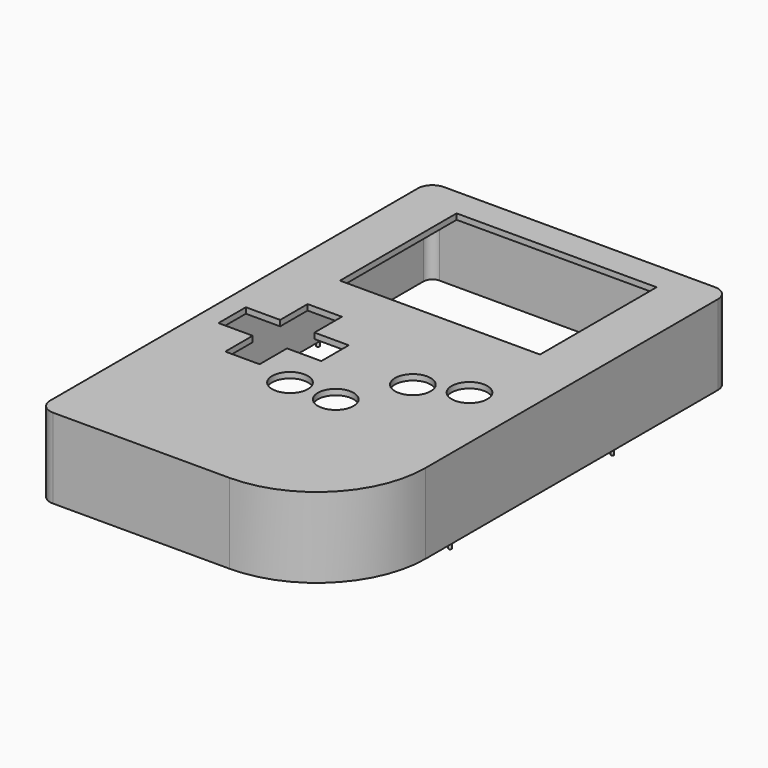
from build123d import *

# Parameters (mm, degrees)
F0_W         = 105
F0_H         = 171
F1_DEPTH     = 28
F3_R         = 38.1
F4_R         = 5.08
F5_T         = -2
F2_W         = 70
F2_H         = 51
F2_R         = 6.25
F6_DEPTH     = 2
F7_TEXT_SIZE = 7.9061016953
F8_DEPTH     = 1
F9_R         = 0.5
F10_DEPTH    = 2


# Not quite as in the source:
# - Text() gives the source's letters only with a copy of the font that has no kerning and outlines rounded to 1/6400 em; it was checked with that copy


with BuildPart() as f1:
    # F0 (on Top) → F1 (new body)
    with BuildSketch(Plane.XY):
        with Locations((52.5, 85.5)):
            Rectangle(F0_W, F0_H)
    extrude(amount=F1_DEPTH)

    # F3
    f3_edges = [f1.edges().sort_by_distance(p)[0] for p in [
        (105, 0, 14),
    ]]
    fillet(f3_edges, radius=F3_R)

    # F4
    f4_edges = [f1.edges().sort_by_distance(p)[0] for p in [
        (0, 0, 14),
        (0, 171, 14),
        (105, 171, 14),
    ]]
    fillet(f4_edges, radius=F4_R)

    # F5
    f5_openings = [f1.faces().sort_by_distance(p)[0] for p in [
        (51.738712, 86.834126, 0),
    ]]
    offset(amount=F5_T, openings=f5_openings)

    # F2 (on face) → F6 (cut, through all)
    with BuildSketch(Plane.XY.offset(28)):
        with Locations((52.5, 135.5)):
            Rectangle(F2_W, F2_H)
        Polygon((19.25, 81.6398638973), (7.25, 81.6398638973), (7.25, 69.6398638973), (19.25, 69.6398638973), (19.25, 57.6398638973), (31.25, 57.6398638973), (31.25, 69.6398638973), (43.25, 69.6398638973), (43.25, 81.6398638973), (31.25, 81.6398638973), (31.25, 93.6398638973), (19.25, 93.6398638973), align=None)
        with Locations((86.5, 80.3898638973)):
            Circle(F2_R)
        with Locations((71.5, 74.3898638973)):
            Circle(F2_R)
        with Locations((44.5, 54.3898638973)):
            Circle(F2_R)
        with Locations((60.5, 54.3898638973)):
            Circle(F2_R)
    extrude(amount=-F6_DEPTH, mode=Mode.SUBTRACT)

    # F7 (on face) → F8 (cut)
    with BuildSketch(Plane(origin=(0, 0, 26), x_dir=(1, 0, 0), z_dir=(0, 0, -1))):
        with Locations((2, -18.2658384198)):
            Text('Jane is rad', F7_TEXT_SIZE, font='Arimo', text_align=(TextAlign.LEFT, TextAlign.BOTTOM))
    extrude(amount=-F8_DEPTH, mode=Mode.SUBTRACT)

    # F9 (on face) → F10 (join)
    with BuildSketch(Plane.XY):
        with Locations((104, 50)):
            Circle(F9_R)
        with Locations((1, 50)):
            Circle(F9_R)
        with Locations((1, 121)):
            Circle(F9_R)
        with Locations((104, 121)):
            Circle(F9_R)
    extrude(amount=-F10_DEPTH)


solid = f1.part
